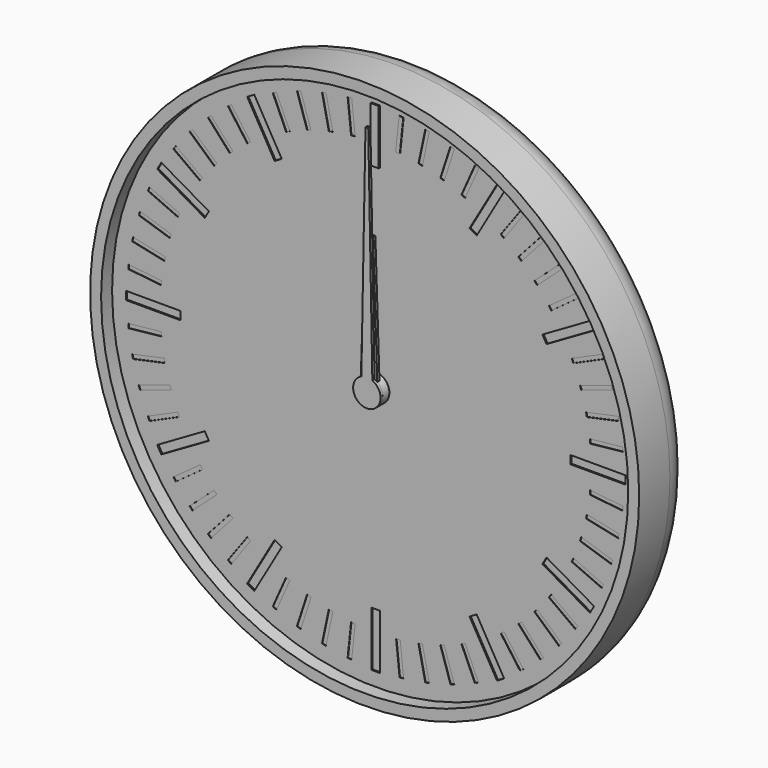
from build123d import *

# Parameters (mm, degrees)
F0_R      = 100
F1_DEPTH  = 24
F2_R      = 10
F3_T      = -4
F4_R      = 5
F4_R_2    = 3
F5_DEPTH  = 2
F6_DEPTH  = 19
F7_DEPTH  = 8
F9_DEPTH  = 4
F11_DEPTH = 4
F12_R     = 5
F12_R_2   = 3
F13_DEPTH = 2
F14_R     = 3
F15_DEPTH = 4
F17_DEPTH = 4
F18_R     = 3
F19_DEPTH = 2
F20_R     = 98
F20_R_2   = 5
F21_DEPTH = 1
F23_R     = 5
F23_R_2   = 3
F24_DEPTH = 2
F25_W     = 3
F25_H     = 20
F25_W_2   = 20
F25_H_2   = 3
F26_DEPTH = 0.5
F27_W     = 1.5
F27_H     = 12
F27_W_2   = 12
F27_H_2   = 1.5
F28_DEPTH = 0.2
F29_DEPTH = 1
F30_DEPTH = 0.4
F31_R     = 5
F31_R_2   = 3
F32_DEPTH = 5
F33_R     = 3
F34_DEPTH = 1
F36_DEPTH = 1


with BuildPart() as f1:
    # F0 (on Front) → F1 (new body)
    with BuildSketch(Plane.XZ):
        Circle(F0_R)
    extrude(amount=F1_DEPTH)

    # F2
    f2_edges = [f1.edges().sort_by_distance(p)[0] for p in [
        (-100, 0, 0),
    ]]
    fillet(f2_edges, radius=F2_R)

    # F3
    f3_openings = [f1.faces().sort_by_distance(p)[0] for p in [
        (0, -24, 0),
    ]]
    offset(amount=F3_T, openings=f3_openings)

    # F4 (on face) → F5 (join)
    with BuildSketch(Plane.XZ.offset(4)):
        Circle(F4_R)
        Circle(F4_R_2, mode=Mode.SUBTRACT)
        with Locations((40, 0)):
            Circle(F4_R)
        with Locations((40, 0)):
            Circle(F4_R_2, mode=Mode.SUBTRACT)
    extrude(amount=F5_DEPTH)


with BuildPart() as f6:
    # F6 (new): a face of the model
    f6_faces = [f1.part.faces().sort_by_distance(p)[0] for p in [
        (0, -4, 0),
    ]]
    extrude(f6_faces, amount=F6_DEPTH)

    # F8 (on face) → F9 (join)
    with BuildSketch(Plane.XZ.offset(6)):
        with BuildLine():
            ThreePointArc((9.2729637667, -1.3794085621), (9.3494561423, -0.6915886375), (9.375, 0))
            ThreePointArc((9.375, 0), (9.3494561423, 0.6915886375), (9.2729637667, 1.3794085621))
            ThreePointArc((9.2729637667, 1.3794085621), (8.9161548403, 2.8970343223), (8.3127812852, 4.3345463782))
            ThreePointArc((8.3127812852, 4.3345463782), (7.5845343223, 5.5104867402), (6.6911892658, 6.566476316))
            ThreePointArc((6.6911892658, 6.566476316), (5.5104867402, 7.5845343223), (4.1773988938, 8.3928519278))
            ThreePointArc((4.1773988938, 8.3928519278), (2.8970343223, 8.9161548403), (1.5536078905, 9.2453733036))
            ThreePointArc((1.5536078905, 9.2453733036), (0, 9.375), (-1.5536078905, 9.2453733036))
            ThreePointArc((-1.5536078905, 9.2453733036), (-2.8970343223, 8.9161548403), (-4.1773988938, 8.3928519278))
            ThreePointArc((-4.1773988938, 8.3928519278), (-5.5104867402, 7.5845343223), (-6.6911892658, 6.566476316))
            ThreePointArc((-6.6911892658, 6.566476316), (-7.5845343223, 5.5104867402), (-8.3127812852, 4.3345463782))
            ThreePointArc((-8.3127812852, 4.3345463782), (-8.9161548403, 2.8970343223), (-9.2729637667, 1.3794085621))
            ThreePointArc((-9.2729637667, 1.3794085621), (-9.375, 0), (-9.2729637667, -1.3794085621))
            ThreePointArc((-9.2729637667, -1.3794085621), (-8.9161548403, -2.8970343223), (-8.3127812852, -4.3345463782))
            ThreePointArc((-8.3127812852, -4.3345463782), (-7.5845343223, -5.5104867402), (-6.6911892658, -6.566476316))
            ThreePointArc((-6.6911892658, -6.566476316), (-5.5104867402, -7.5845343223), (-4.1773988938, -8.3928519278))
            ThreePointArc((-4.1773988938, -8.3928519278), (-2.8970343223, -8.9161548403), (-1.5536078905, -9.2453733036))
            ThreePointArc((-1.5536078905, -9.2453733036), (0, -9.375), (1.5536078905, -9.2453733036))
            ThreePointArc((1.5536078905, -9.2453733036), (2.8970343223, -8.9161548403), (4.1773988938, -8.3928519278))
            ThreePointArc((4.1773988938, -8.3928519278), (5.5104867402, -7.5845343223), (6.6911892658, -6.566476316))
            ThreePointArc((6.6911892658, -6.566476316), (7.5845343223, -5.5104867402), (8.3127812852, -4.3345463782))
            ThreePointArc((8.3127812852, -4.3345463782), (8.9161548403, -2.8970343223), (9.2729637667, -1.3794085621))
        make_face()
        with BuildLine():
            ThreePointArc((8.3127812852, 4.3345463782), (8.9161548403, 2.8970343223), (9.2729637667, 1.3794085621))
            Line((9.2729637667, 1.3794085621), (11.1823199426, 2.3946312492))
            Line((11.1823199426, 2.3946312492), (10.8182678729, 3.515068311))
            Line((10.8182678729, 3.515068311), (10.4542158031, 4.6355053728))
            Line((10.4542158031, 4.6355053728), (8.3127812852, 4.3345463782))
        make_face()
        with BuildLine():
            Line((11.1823199426, -2.3946312492), (9.2729637667, -1.3794085621))
            ThreePointArc((9.2729637667, -1.3794085621), (8.9161548403, -2.8970343223), (8.3127812852, -4.3345463782))
            Line((8.3127812852, -4.3345463782), (10.4542158031, -4.6355053728))
            Line((10.4542158031, -4.6355053728), (10.8182678729, -3.515068311))
            Line((10.8182678729, -3.515068311), (11.1823199426, -2.3946312492))
        make_face()
        with BuildLine():
            ThreePointArc((4.1773988938, 8.3928519278), (5.5104867402, 7.5845343223), (6.6911892658, 6.566476316))
            Line((6.6911892658, 6.566476316), (7.6391579371, 8.5101001246))
            Line((7.6391579371, 8.5101001246), (6.6860572448, 9.202568311))
            Line((6.6860572448, 9.202568311), (5.7329565525, 9.8950364974))
            Line((5.7329565525, 9.8950364974), (4.1773988938, 8.3928519278))
        make_face()
        with BuildLine():
            Line((7.6391579371, -8.5101001246), (6.6911892658, -6.566476316))
            ThreePointArc((6.6911892658, -6.566476316), (5.5104867402, -7.5845343223), (4.1773988938, -8.3928519278))
            Line((4.1773988938, -8.3928519278), (5.7329565525, -9.8950364974))
            Line((5.7329565525, -9.8950364974), (6.6860572448, -9.202568311))
            Line((6.6860572448, -9.202568311), (7.6391579371, -8.5101001246))
        make_face()
        with BuildLine():
            ThreePointArc((-1.5536078905, 9.2453733036), (0, 9.375), (1.5536078905, 9.2453733036))
            Line((1.5536078905, 9.2453733036), (1.1780972451, 11.375))
            Line((1.1780972451, 11.375), (0, 11.375))
            Line((0, 11.375), (-1.1780972451, 11.375))
            Line((-1.1780972451, 11.375), (-1.5536078905, 9.2453733036))
        make_face()
        with BuildLine():
            Line((1.1780972451, -11.375), (1.5536078905, -9.2453733036))
            ThreePointArc((1.5536078905, -9.2453733036), (0, -9.375), (-1.5536078905, -9.2453733036))
            Line((-1.5536078905, -9.2453733036), (-1.1780972451, -11.375))
            Line((-1.1780972451, -11.375), (0, -11.375))
            Line((0, -11.375), (1.1780972451, -11.375))
        make_face()
        with BuildLine():
            ThreePointArc((-6.6911892658, 6.566476316), (-5.5104867402, 7.5845343223), (-4.1773988938, 8.3928519278))
            Line((-4.1773988938, 8.3928519278), (-5.7329565525, 9.8950364974))
            Line((-5.7329565525, 9.8950364974), (-6.6860572448, 9.202568311))
            Line((-6.6860572448, 9.202568311), (-7.6391579371, 8.5101001246))
            Line((-7.6391579371, 8.5101001246), (-6.6911892658, 6.566476316))
        make_face()
        with BuildLine():
            Line((-5.7329565525, -9.8950364974), (-4.1773988938, -8.3928519278))
            ThreePointArc((-4.1773988938, -8.3928519278), (-5.5104867402, -7.5845343223), (-6.6911892658, -6.566476316))
            Line((-6.6911892658, -6.566476316), (-7.6391579371, -8.5101001246))
            Line((-7.6391579371, -8.5101001246), (-6.6860572448, -9.202568311))
            Line((-6.6860572448, -9.202568311), (-5.7329565525, -9.8950364974))
        make_face()
        with BuildLine():
            ThreePointArc((-9.2729637667, 1.3794085621), (-8.9161548403, 2.8970343223), (-8.3127812852, 4.3345463782))
            Line((-8.3127812852, 4.3345463782), (-10.4542158031, 4.6355053728))
            Line((-10.4542158031, 4.6355053728), (-10.8182678729, 3.515068311))
            Line((-10.8182678729, 3.515068311), (-11.1823199426, 2.3946312492))
            Line((-11.1823199426, 2.3946312492), (-9.2729637667, 1.3794085621))
        make_face()
        with BuildLine():
            Line((-10.4542158031, -4.6355053728), (-8.3127812852, -4.3345463782))
            ThreePointArc((-8.3127812852, -4.3345463782), (-8.9161548403, -2.8970343223), (-9.2729637667, -1.3794085621))
            Line((-9.2729637667, -1.3794085621), (-11.1823199426, -2.3946312492))
            Line((-11.1823199426, -2.3946312492), (-10.8182678729, -3.515068311))
            Line((-10.8182678729, -3.515068311), (-10.4542158031, -4.6355053728))
        make_face()
    extrude(amount=F9_DEPTH)

    # F35 (on face) → F36 (join)
    with BuildSketch(Plane.XZ.offset(23)):
        with BuildLine():
            ThreePointArc((-2, 4.582575695), (-2.7386127875, -4.1833001327), (5, 0))
            ThreePointArc((5, 0), (4.1833001327, 2.7386127875), (2, 4.582575695))
            ThreePointArc((2, 4.582575695), (0, 5), (-2, 4.582575695))
        make_face()
        with BuildLine():
            ThreePointArc((-2, 4.582575695), (0, 5), (2, 4.582575695))
            Line((2, 4.582575695), (0.5, 85))
            Line((0.5, 85), (0, 85))
            Line((0, 85), (-0.5, 85))
            Line((-0.5, 85), (-2, 4.582575695))
        make_face()
    extrude(amount=-F36_DEPTH)


with BuildPart() as f7:
    # F7 (new): a face of the model
    f7_faces = [f1.part.faces().sort_by_distance(p)[0] for p in [
        (40, -4, 0),
    ]]
    extrude(f7_faces, amount=F7_DEPTH)

    # F10 (on face) → F11 (join)
    with BuildSketch(Plane.XZ.offset(6)):
        with BuildLine():
            ThreePointArc((68.0829066802, -1.5381733945), (68.1144747006, -0.7693746225), (68.125, 0))
            ThreePointArc((68.125, 0), (68.1144747006, 0.7693746225), (68.0829066802, 1.5381733945))
            ThreePointArc((68.0829066802, 1.5381733945), (67.9709283072, 2.9398630294), (67.7890320221, 4.3342039956))
            ThreePointArc((67.7890320221, 4.3342039956), (67.5104012706, 5.8475163042), (67.1494235596, 7.3433252263))
            ThreePointArc((67.1494235596, 7.3433252263), (66.7484645208, 8.6911029668), (66.280643318, 10.0171558733))
            ThreePointArc((66.280643318, 10.0171558733), (65.6934659962, 11.4394680865), (65.0293803521, 12.8275385085))
            ThreePointArc((65.0293803521, 12.8275385085), (64.3569644814, 14.0625), (63.6236643925, 15.2623099717))
            ThreePointArc((63.6236643925, 15.2623099717), (62.7536029668, 16.5314602207), (61.815433119, 17.7511268046))
            ThreePointArc((61.815433119, 17.7511268046), (60.9009482166, 18.8192983038), (59.934217974, 19.8404278876))
            ThreePointArc((59.934217974, 19.8404278876), (58.8192983038, 20.9009482166), (57.6480467764, 21.8989056799))
            ThreePointArc((57.6480467764, 21.8989056799), (56.5314602207, 22.7536029668), (55.3735505752, 23.5514238999))
            ThreePointArc((55.3735505752, 23.5514238999), (54.0625, 24.3569644814), (52.709356105, 25.0895972944))
            ThreePointArc((52.709356105, 25.0895972944), (51.4394680865, 25.6934659962), (50.1409852457, 26.2331096755))
            ThreePointArc((50.1409852457, 26.2331096755), (48.6911029668, 26.7484645208), (47.2152055856, 27.1837531139))
            ThreePointArc((47.2152055856, 27.1837531139), (45.8475163042, 27.5104012706), (44.4652101991, 27.7682826779))
            ThreePointArc((44.4652101991, 27.7682826779), (42.9398630294, 27.9709283072), (41.4057159597, 28.0898484802))
            ThreePointArc((41.4057159597, 28.0898484802), (40, 28.125), (38.5942840403, 28.0898484802))
            ThreePointArc((38.5942840403, 28.0898484802), (37.0601369706, 27.9709283072), (35.5347898009, 27.7682826779))
            ThreePointArc((35.5347898009, 27.7682826779), (34.1524836958, 27.5104012706), (32.7847944144, 27.1837531139))
            ThreePointArc((32.7847944144, 27.1837531139), (31.3088970332, 26.7484645208), (29.8590147543, 26.2331096755))
            ThreePointArc((29.8590147543, 26.2331096755), (28.5605319135, 25.6934659962), (27.290643895, 25.0895972944))
            ThreePointArc((27.290643895, 25.0895972944), (25.9375, 24.3569644814), (24.6264494248, 23.5514238999))
            ThreePointArc((24.6264494248, 23.5514238999), (23.4685397793, 22.7536029668), (22.3519532236, 21.8989056799))
            ThreePointArc((22.3519532236, 21.8989056799), (21.1807016962, 20.9009482166), (20.065782026, 19.8404278876))
            ThreePointArc((20.065782026, 19.8404278876), (19.0990517834, 18.8192983038), (18.184566881, 17.7511268046))
            ThreePointArc((18.184566881, 17.7511268046), (17.2463970332, 16.5314602207), (16.3763356075, 15.2623099717))
            ThreePointArc((16.3763356075, 15.2623099717), (15.6430355186, 14.0625), (14.9706196479, 12.8275385085))
            ThreePointArc((14.9706196479, 12.8275385085), (14.3065340038, 11.4394680865), (13.719356682, 10.0171558733))
            ThreePointArc((13.719356682, 10.0171558733), (13.2515354792, 8.6911029668), (12.8505764404, 7.3433252263))
            ThreePointArc((12.8505764404, 7.3433252263), (12.4895987294, 5.8475163042), (12.2109679779, 4.3342039956))
            ThreePointArc((12.2109679779, 4.3342039956), (12.0290716928, 2.9398630294), (11.9170933198, 1.5381733945))
            ThreePointArc((11.9170933198, 1.5381733945), (11.875, 0), (11.9170933198, -1.5381733945))
            ThreePointArc((11.9170933198, -1.5381733945), (12.0290716928, -2.9398630294), (12.2109679779, -4.3342039956))
            ThreePointArc((12.2109679779, -4.3342039956), (12.4895987294, -5.8475163042), (12.8505764404, -7.3433252263))
            ThreePointArc((12.8505764404, -7.3433252263), (13.2515354792, -8.6911029668), (13.719356682, -10.0171558733))
            ThreePointArc((13.719356682, -10.0171558733), (14.3065340038, -11.4394680865), (14.9706196479, -12.8275385085))
            ThreePointArc((14.9706196479, -12.8275385085), (15.6430355186, -14.0625), (16.3763356075, -15.2623099717))
            ThreePointArc((16.3763356075, -15.2623099717), (17.2463970332, -16.5314602207), (18.184566881, -17.7511268046))
            ThreePointArc((18.184566881, -17.7511268046), (19.0990517834, -18.8192983038), (20.065782026, -19.8404278876))
            ThreePointArc((20.065782026, -19.8404278876), (21.1807016962, -20.9009482166), (22.3519532236, -21.8989056799))
            ThreePointArc((22.3519532236, -21.8989056799), (23.4685397793, -22.7536029668), (24.6264494248, -23.5514238999))
            ThreePointArc((24.6264494248, -23.5514238999), (25.9375, -24.3569644814), (27.290643895, -25.0895972944))
            ThreePointArc((27.290643895, -25.0895972944), (28.5605319135, -25.6934659962), (29.8590147543, -26.2331096755))
            ThreePointArc((29.8590147543, -26.2331096755), (31.3088970332, -26.7484645208), (32.7847944144, -27.1837531139))
            ThreePointArc((32.7847944144, -27.1837531139), (34.1524836958, -27.5104012706), (35.5347898009, -27.7682826779))
            ThreePointArc((35.5347898009, -27.7682826779), (37.0601369706, -27.9709283072), (38.5942840403, -28.0898484802))
            ThreePointArc((38.5942840403, -28.0898484802), (40, -28.125), (41.4057159597, -28.0898484802))
            ThreePointArc((41.4057159597, -28.0898484802), (42.9398630294, -27.9709283072), (44.4652101991, -27.7682826779))
            ThreePointArc((44.4652101991, -27.7682826779), (45.8475163042, -27.5104012706), (47.2152055856, -27.1837531139))
            ThreePointArc((47.2152055856, -27.1837531139), (48.6911029668, -26.7484645208), (50.1409852457, -26.2331096755))
            ThreePointArc((50.1409852457, -26.2331096755), (51.4394680865, -25.6934659962), (52.709356105, -25.0895972944))
            ThreePointArc((52.709356105, -25.0895972944), (54.0625, -24.3569644814), (55.3735505752, -23.5514238999))
            ThreePointArc((55.3735505752, -23.5514238999), (56.5314602207, -22.7536029668), (57.6480467764, -21.8989056799))
            ThreePointArc((57.6480467764, -21.8989056799), (58.8192983038, -20.9009482166), (59.934217974, -19.8404278876))
            ThreePointArc((59.934217974, -19.8404278876), (60.9009482166, -18.8192983038), (61.815433119, -17.7511268046))
            ThreePointArc((61.815433119, -17.7511268046), (62.7536029668, -16.5314602207), (63.6236643925, -15.2623099717))
            ThreePointArc((63.6236643925, -15.2623099717), (64.3569644814, -14.0625), (65.0293803521, -12.8275385085))
            ThreePointArc((65.0293803521, -12.8275385085), (65.6934659962, -11.4394680865), (66.280643318, -10.0171558733))
            ThreePointArc((66.280643318, -10.0171558733), (66.7484645208, -8.6911029668), (67.1494235596, -7.3433252263))
            ThreePointArc((67.1494235596, -7.3433252263), (67.5104012706, -5.8475163042), (67.7890320221, -4.3342039956))
            ThreePointArc((67.7890320221, -4.3342039956), (67.9709283072, -2.9398630294), (68.0829066802, -1.5381733945))
        make_face()
        with BuildLine():
            ThreePointArc((68.0829066802, 1.5381733945), (68.1144747006, 0.7693746225), (68.125, 0))
            ThreePointArc((68.125, 0), (68.1144747006, -0.7693746225), (68.0829066802, -1.5381733945))
            Line((68.0829066802, -1.5381733945), (70.125, -1.1780972451))
            Line((70.125, -1.1780972451), (70.125, 0))
            Line((70.125, 0), (70.125, 1.1780972451))
            Line((70.125, 1.1780972451), (68.0829066802, 1.5381733945))
        make_face()
        with BuildLine():
            ThreePointArc((67.1494235596, 7.3433252263), (67.5104012706, 5.8475163042), (67.7890320221, 4.3342039956))
            Line((67.7890320221, 4.3342039956), (69.7116366623, 5.1109866922))
            Line((69.7116366623, 5.1109866922), (69.4666964721, 6.2633396859))
            Line((69.4666964721, 6.2633396859), (69.2217562819, 7.4156926796))
            Line((69.2217562819, 7.4156926796), (67.1494235596, 7.3433252263))
        make_face()
        with BuildLine():
            Line((69.7116366623, -5.1109866922), (67.7890320221, -4.3342039956))
            ThreePointArc((67.7890320221, -4.3342039956), (67.5104012706, -5.8475163042), (67.1494235596, -7.3433252263))
            Line((67.1494235596, -7.3433252263), (69.2217562819, -7.4156926796))
            Line((69.2217562819, -7.4156926796), (69.4666964721, -6.2633396859))
            Line((69.4666964721, -6.2633396859), (69.7116366623, -5.1109866922))
        make_face()
        with BuildLine():
            ThreePointArc((65.0293803521, 12.8275385085), (65.6934659962, 11.4394680865), (66.280643318, 10.0171558733))
            Line((66.280643318, 10.0171558733), (67.9997322302, 11.1766959857))
            Line((67.9997322302, 11.1766959857), (67.5205569115, 12.2529413727))
            Line((67.5205569115, 12.2529413727), (67.0413815928, 13.3291867596))
            Line((67.0413815928, 13.3291867596), (65.0293803521, 12.8275385085))
        make_face()
        with BuildLine():
            Line((67.9997322302, -11.1766959857), (66.280643318, -10.0171558733))
            ThreePointArc((66.280643318, -10.0171558733), (65.6934659962, -11.4394680865), (65.0293803521, -12.8275385085))
            Line((65.0293803521, -12.8275385085), (67.0413815928, -13.3291867596))
            Line((67.0413815928, -13.3291867596), (67.5205569115, -12.2529413727))
            Line((67.5205569115, -12.2529413727), (67.9997322302, -11.1766959857))
        make_face()
        with BuildLine():
            ThreePointArc((61.815433119, 17.7511268046), (62.7536029668, 16.5314602207), (63.6236643925, 15.2623099717))
            Line((63.6236643925, 15.2623099717), (65.064105142, 16.753930033))
            Line((65.064105142, 16.753930033), (64.3716369555, 17.7070307253))
            Line((64.3716369555, 17.7070307253), (63.6791687691, 18.6601314176))
            Line((63.6791687691, 18.6601314176), (61.815433119, 17.7511268046))
        make_face()
        with BuildLine():
            Line((65.064105142, -16.753930033), (63.6236643925, -15.2623099717))
            ThreePointArc((63.6236643925, -15.2623099717), (62.7536029668, -16.5314602207), (61.815433119, -17.7511268046))
            Line((61.815433119, -17.7511268046), (63.6791687691, -18.6601314176))
            Line((63.6791687691, -18.6601314176), (64.3716369555, -17.7070307253))
            Line((64.3716369555, -17.7070307253), (65.064105142, -16.753930033))
        make_face()
        with BuildLine():
            ThreePointArc((57.6480467764, 21.8989056799), (58.8192983038, 20.9009482166), (59.934217974, 19.8404278876))
            Line((59.934217974, 19.8404278876), (61.0330563882, 21.5989369435))
            Line((61.0330563882, 21.5989369435), (60.1575595166, 22.3872378675))
            Line((60.1575595166, 22.3872378675), (59.282062645, 23.1755387915))
            Line((59.282062645, 23.1755387915), (57.6480467764, 21.8989056799))
        make_face()
        with BuildLine():
            Line((61.0330563882, -21.5989369435), (59.934217974, -19.8404278876))
            ThreePointArc((59.934217974, -19.8404278876), (58.8192983038, -20.9009482166), (57.6480467764, -21.8989056799))
            Line((57.6480467764, -21.8989056799), (59.282062645, -23.1755387915))
            Line((59.282062645, -23.1755387915), (60.1575595166, -22.3872378675))
            Line((60.1575595166, -22.3872378675), (61.0330563882, -21.5989369435))
        make_face()
        with BuildLine():
            ThreePointArc((52.709356105, 25.0895972944), (54.0625, 24.3569644814), (55.3735505752, 23.5514238999))
            Line((55.3735505752, 23.5514238999), (56.0827621424, 25.4999666665))
            Line((56.0827621424, 25.4999666665), (55.0625, 26.089015289))
            Line((55.0625, 26.089015289), (54.0422378576, 26.6780639116))
            Line((54.0422378576, 26.6780639116), (52.709356105, 25.0895972944))
        make_face()
        with BuildLine():
            Line((56.0827621424, -25.4999666665), (55.3735505752, -23.5514238999))
            ThreePointArc((55.3735505752, -23.5514238999), (54.0625, -24.3569644814), (52.709356105, -25.0895972944))
            Line((52.709356105, -25.0895972944), (54.0422378576, -26.6780639116))
            Line((54.0422378576, -26.6780639116), (55.0625, -26.089015289))
            Line((55.0625, -26.089015289), (56.0827621424, -25.4999666665))
        make_face()
        with BuildLine():
            ThreePointArc((47.2152055856, 27.1837531139), (48.6911029668, 26.7484645208), (50.1409852457, 26.2331096755))
            Line((50.1409852457, 26.2331096755), (50.4295740173, 28.2865254836))
            Line((50.4295740173, 28.2865254836), (49.3091369555, 28.6505775534))
            Line((49.3091369555, 28.6505775534), (48.1886998938, 29.0146296232))
            Line((48.1886998938, 29.0146296232), (47.2152055856, 27.1837531139))
        make_face()
        with BuildLine():
            Line((50.4295740173, -28.2865254836), (50.1409852457, -26.2331096755))
            ThreePointArc((50.1409852457, -26.2331096755), (48.6911029668, -26.7484645208), (47.2152055856, -27.1837531139))
            Line((47.2152055856, -27.1837531139), (48.1886998938, -29.0146296232))
            Line((48.1886998938, -29.0146296232), (49.3091369555, -28.6505775534))
            Line((49.3091369555, -28.6505775534), (50.4295740173, -28.2865254836))
        make_face()
        with BuildLine():
            ThreePointArc((41.4057159597, 28.0898484802), (42.9398630294, 27.9709283072), (44.4652101991, 27.7682826779))
            Line((44.4652101991, 27.7682826779), (44.3205634611, 29.8368274034))
            Line((44.3205634611, 29.8368274034), (43.1489199559, 29.959972098))
            Line((43.1489199559, 29.959972098), (41.9772764508, 30.0831167926))
            Line((41.9772764508, 30.0831167926), (41.4057159597, 28.0898484802))
        make_face()
        with BuildLine():
            Line((44.3205634611, -29.8368274034), (44.4652101991, -27.7682826779))
            ThreePointArc((44.4652101991, -27.7682826779), (42.9398630294, -27.9709283072), (41.4057159597, -28.0898484802))
            Line((41.4057159597, -28.0898484802), (41.9772764508, -30.0831167926))
            Line((41.9772764508, -30.0831167926), (43.1489199559, -29.959972098))
            Line((43.1489199559, -29.959972098), (44.3205634611, -29.8368274034))
        make_face()
        with BuildLine():
            ThreePointArc((35.5347898009, 27.7682826779), (37.0601369706, 27.9709283072), (38.5942840403, 28.0898484802))
            Line((38.5942840403, 28.0898484802), (38.0227235492, 30.0831167926))
            Line((38.0227235492, 30.0831167926), (36.8510800441, 29.959972098))
            Line((36.8510800441, 29.959972098), (35.6794365389, 29.8368274034))
            Line((35.6794365389, 29.8368274034), (35.5347898009, 27.7682826779))
        make_face()
        with BuildLine():
            Line((38.0227235492, -30.0831167926), (38.5942840403, -28.0898484802))
            ThreePointArc((38.5942840403, -28.0898484802), (37.0601369706, -27.9709283072), (35.5347898009, -27.7682826779))
            Line((35.5347898009, -27.7682826779), (35.6794365389, -29.8368274034))
            Line((35.6794365389, -29.8368274034), (36.8510800441, -29.959972098))
            Line((36.8510800441, -29.959972098), (38.0227235492, -30.0831167926))
        make_face()
        with BuildLine():
            ThreePointArc((29.8590147543, 26.2331096755), (31.3088970332, 26.7484645208), (32.7847944144, 27.1837531139))
            Line((32.7847944144, 27.1837531139), (31.8113001062, 29.0146296232))
            Line((31.8113001062, 29.0146296232), (30.6908630445, 28.6505775534))
            Line((30.6908630445, 28.6505775534), (29.5704259827, 28.2865254836))
            Line((29.5704259827, 28.2865254836), (29.8590147543, 26.2331096755))
        make_face()
        with BuildLine():
            Line((31.8113001062, -29.0146296232), (32.7847944144, -27.1837531139))
            ThreePointArc((32.7847944144, -27.1837531139), (31.3088970332, -26.7484645208), (29.8590147543, -26.2331096755))
            Line((29.8590147543, -26.2331096755), (29.5704259827, -28.2865254836))
            Line((29.5704259827, -28.2865254836), (30.6908630445, -28.6505775534))
            Line((30.6908630445, -28.6505775534), (31.8113001062, -29.0146296232))
        make_face()
        with BuildLine():
            ThreePointArc((24.6264494248, 23.5514238999), (25.9375, 24.3569644814), (27.290643895, 25.0895972944))
            Line((27.290643895, 25.0895972944), (25.9577621424, 26.6780639116))
            Line((25.9577621424, 26.6780639116), (24.9375, 26.089015289))
            Line((24.9375, 26.089015289), (23.9172378576, 25.4999666665))
            Line((23.9172378576, 25.4999666665), (24.6264494248, 23.5514238999))
        make_face()
        with BuildLine():
            Line((25.9577621424, -26.6780639116), (27.290643895, -25.0895972944))
            ThreePointArc((27.290643895, -25.0895972944), (25.9375, -24.3569644814), (24.6264494248, -23.5514238999))
            Line((24.6264494248, -23.5514238999), (23.9172378576, -25.4999666665))
            Line((23.9172378576, -25.4999666665), (24.9375, -26.089015289))
            Line((24.9375, -26.089015289), (25.9577621424, -26.6780639116))
        make_face()
        with BuildLine():
            ThreePointArc((20.065782026, 19.8404278876), (21.1807016962, 20.9009482166), (22.3519532236, 21.8989056799))
            Line((22.3519532236, 21.8989056799), (20.717937355, 23.1755387915))
            Line((20.717937355, 23.1755387915), (19.8424404834, 22.3872378675))
            Line((19.8424404834, 22.3872378675), (18.9669436118, 21.5989369435))
            Line((18.9669436118, 21.5989369435), (20.065782026, 19.8404278876))
        make_face()
        with BuildLine():
            Line((20.717937355, -23.1755387915), (22.3519532236, -21.8989056799))
            ThreePointArc((22.3519532236, -21.8989056799), (21.1807016962, -20.9009482166), (20.065782026, -19.8404278876))
            Line((20.065782026, -19.8404278876), (18.9669436118, -21.5989369435))
            Line((18.9669436118, -21.5989369435), (19.8424404834, -22.3872378675))
            Line((19.8424404834, -22.3872378675), (20.717937355, -23.1755387915))
        make_face()
        with BuildLine():
            ThreePointArc((16.3763356075, 15.2623099717), (17.2463970332, 16.5314602207), (18.184566881, 17.7511268046))
            Line((18.184566881, 17.7511268046), (16.3208312309, 18.6601314176))
            Line((16.3208312309, 18.6601314176), (15.6283630445, 17.7070307253))
            Line((15.6283630445, 17.7070307253), (14.935894858, 16.753930033))
            Line((14.935894858, 16.753930033), (16.3763356075, 15.2623099717))
        make_face()
        with BuildLine():
            Line((16.3208312309, -18.6601314176), (18.184566881, -17.7511268046))
            ThreePointArc((18.184566881, -17.7511268046), (17.2463970332, -16.5314602207), (16.3763356075, -15.2623099717))
            Line((16.3763356075, -15.2623099717), (14.935894858, -16.753930033))
            Line((14.935894858, -16.753930033), (15.6283630445, -17.7070307253))
            Line((15.6283630445, -17.7070307253), (16.3208312309, -18.6601314176))
        make_face()
        with BuildLine():
            ThreePointArc((13.719356682, 10.0171558733), (14.3065340038, 11.4394680865), (14.9706196479, 12.8275385085))
            Line((14.9706196479, 12.8275385085), (12.9586184072, 13.3291867596))
            Line((12.9586184072, 13.3291867596), (12.4794430885, 12.2529413727))
            Line((12.4794430885, 12.2529413727), (12.0002677698, 11.1766959857))
            Line((12.0002677698, 11.1766959857), (13.719356682, 10.0171558733))
        make_face()
        with BuildLine():
            Line((12.9586184072, -13.3291867596), (14.9706196479, -12.8275385085))
            ThreePointArc((14.9706196479, -12.8275385085), (14.3065340038, -11.4394680865), (13.719356682, -10.0171558733))
            Line((13.719356682, -10.0171558733), (12.0002677698, -11.1766959857))
            Line((12.0002677698, -11.1766959857), (12.4794430885, -12.2529413727))
            Line((12.4794430885, -12.2529413727), (12.9586184072, -13.3291867596))
        make_face()
        with BuildLine():
            ThreePointArc((12.2109679779, 4.3342039956), (12.4895987294, 5.8475163042), (12.8505764404, 7.3433252263))
            Line((12.8505764404, 7.3433252263), (10.7782437181, 7.4156926796))
            Line((10.7782437181, 7.4156926796), (10.5333035279, 6.2633396859))
            Line((10.5333035279, 6.2633396859), (10.2883633377, 5.1109866922))
            Line((10.2883633377, 5.1109866922), (12.2109679779, 4.3342039956))
        make_face()
        with BuildLine():
            Line((10.7782437181, -7.4156926796), (12.8505764404, -7.3433252263))
            ThreePointArc((12.8505764404, -7.3433252263), (12.4895987294, -5.8475163042), (12.2109679779, -4.3342039956))
            Line((12.2109679779, -4.3342039956), (10.2883633377, -5.1109866922))
            Line((10.2883633377, -5.1109866922), (10.5333035279, -6.2633396859))
            Line((10.5333035279, -6.2633396859), (10.7782437181, -7.4156926796))
        make_face()
        with BuildLine():
            ThreePointArc((11.9170933198, -1.5381733945), (11.875, 0), (11.9170933198, 1.5381733945))
            Line((11.9170933198, 1.5381733945), (9.875, 1.1780972451))
            Line((9.875, 1.1780972451), (9.875, 0))
            Line((9.875, 0), (9.875, -1.1780972451))
            Line((9.875, -1.1780972451), (11.9170933198, -1.5381733945))
        make_face()
    extrude(amount=F11_DEPTH)

    # F16 (on face) → F17 (join)
    with BuildSketch(Plane.XZ.offset(12)):
        with BuildLine():
            ThreePointArc((47.4288750323, -1.0304444454), (47.4821976298, -0.5164480894), (47.5, 0))
            ThreePointArc((47.5, 0), (47.4821976298, 0.5164480894), (47.4288750323, 1.0304444454))
            ThreePointArc((47.4288750323, 1.0304444454), (47.1329238722, 2.3176274578), (46.6157661985, 3.532936117))
            ThreePointArc((46.6157661985, 3.532936117), (46.0676274578, 4.4083893922), (45.4044061018, 5.2002302532))
            ThreePointArc((45.4044061018, 5.2002302532), (44.4083893922, 6.0676274578), (43.2756595386, 6.7468551628))
            ThreePointArc((43.2756595386, 6.7468551628), (42.3176274578, 7.1329238722), (41.3156377295, 7.3837048536))
            ThreePointArc((41.3156377295, 7.3837048536), (40, 7.5), (38.6843622705, 7.3837048536))
            ThreePointArc((38.6843622705, 7.3837048536), (37.6823725422, 7.1329238722), (36.7243404614, 6.7468551628))
            ThreePointArc((36.7243404614, 6.7468551628), (35.5916106078, 6.0676274578), (34.5955938982, 5.2002302532))
            ThreePointArc((34.5955938982, 5.2002302532), (33.9323725422, 4.4083893922), (33.3842338015, 3.532936117))
            ThreePointArc((33.3842338015, 3.532936117), (32.8670761278, 2.3176274578), (32.5711249677, 1.0304444454))
            ThreePointArc((32.5711249677, 1.0304444454), (32.5, 0), (32.5711249677, -1.0304444454))
            ThreePointArc((32.5711249677, -1.0304444454), (32.8670761278, -2.3176274578), (33.3842338015, -3.532936117))
            ThreePointArc((33.3842338015, -3.532936117), (33.9323725422, -4.4083893922), (34.5955938982, -5.2002302532))
            ThreePointArc((34.5955938982, -5.2002302532), (35.5916106078, -6.0676274578), (36.7243404614, -6.7468551628))
            ThreePointArc((36.7243404614, -6.7468551628), (37.6823725422, -7.1329238722), (38.6843622705, -7.3837048536))
            ThreePointArc((38.6843622705, -7.3837048536), (40, -7.5), (41.3156377295, -7.3837048536))
            ThreePointArc((41.3156377295, -7.3837048536), (42.3176274578, -7.1329238722), (43.2756595386, -6.7468551628))
            ThreePointArc((43.2756595386, -6.7468551628), (44.4083893922, -6.0676274578), (45.4044061018, -5.2002302532))
            ThreePointArc((45.4044061018, -5.2002302532), (46.0676274578, -4.4083893922), (46.6157661985, -3.532936117))
            ThreePointArc((46.6157661985, -3.532936117), (47.1329238722, -2.3176274578), (47.4288750323, -1.0304444454))
        make_face()
        with BuildLine():
            ThreePointArc((46.6157661985, 3.532936117), (47.1329238722, 2.3176274578), (47.4288750323, 1.0304444454))
            Line((47.4288750323, 1.0304444454), (49.3262785606, 2.0393117971))
            Line((49.3262785606, 2.0393117971), (48.743795249, 3.832011096))
            Line((48.743795249, 3.832011096), (46.6157661985, 3.532936117))
        make_face()
        with BuildLine():
            Line((49.3262785606, -2.0393117971), (47.4288750323, -1.0304444454))
            ThreePointArc((47.4288750323, -1.0304444454), (47.1329238722, -2.3176274578), (46.6157661985, -3.532936117))
            Line((46.6157661985, -3.532936117), (48.743795249, -3.832011096))
            Line((48.743795249, -3.832011096), (49.3262785606, -2.0393117971))
        make_face()
        with BuildLine():
            ThreePointArc((43.2756595386, 6.7468551628), (44.4083893922, 6.0676274578), (45.4044061018, 5.2002302532))
            Line((45.4044061018, 5.2002302532), (46.3464404506, 7.1316868974))
            Line((46.3464404506, 7.1316868974), (44.8214793429, 8.2396359957))
            Line((44.8214793429, 8.2396359957), (43.2756595386, 6.7468551628))
        make_face()
        with BuildLine():
            Line((46.3464404506, -7.1316868974), (45.4044061018, -5.2002302532))
            ThreePointArc((45.4044061018, -5.2002302532), (44.4083893922, -6.0676274578), (43.2756595386, -6.7468551628))
            Line((43.2756595386, -6.7468551628), (44.8214793429, -8.2396359957))
            Line((44.8214793429, -8.2396359957), (46.3464404506, -7.1316868974))
        make_face()
        with BuildLine():
            ThreePointArc((38.6843622705, 7.3837048536), (40, 7.5), (41.3156377295, 7.3837048536))
            Line((41.3156377295, 7.3837048536), (40.9424777961, 9.5))
            Line((40.9424777961, 9.5), (39.0575222039, 9.5))
            Line((39.0575222039, 9.5), (38.6843622705, 7.3837048536))
        make_face()
        with BuildLine():
            Line((40.9424777961, -9.5), (41.3156377295, -7.3837048536))
            ThreePointArc((41.3156377295, -7.3837048536), (40, -7.5), (38.6843622705, -7.3837048536))
            Line((38.6843622705, -7.3837048536), (39.0575222039, -9.5))
            Line((39.0575222039, -9.5), (40.9424777961, -9.5))
        make_face()
        with BuildLine():
            ThreePointArc((34.5955938982, 5.2002302532), (35.5916106078, 6.0676274578), (36.7243404614, 6.7468551628))
            Line((36.7243404614, 6.7468551628), (35.1785206571, 8.2396359957))
            Line((35.1785206571, 8.2396359957), (33.6535595494, 7.1316868974))
            Line((33.6535595494, 7.1316868974), (34.5955938982, 5.2002302532))
        make_face()
        with BuildLine():
            Line((35.1785206571, -8.2396359957), (36.7243404614, -6.7468551628))
            ThreePointArc((36.7243404614, -6.7468551628), (35.5916106078, -6.0676274578), (34.5955938982, -5.2002302532))
            Line((34.5955938982, -5.2002302532), (33.6535595494, -7.1316868974))
            Line((33.6535595494, -7.1316868974), (35.1785206571, -8.2396359957))
        make_face()
        with BuildLine():
            ThreePointArc((32.5711249677, 1.0304444454), (32.8670761278, 2.3176274578), (33.3842338015, 3.532936117))
            Line((33.3842338015, 3.532936117), (31.256204751, 3.832011096))
            Line((31.256204751, 3.832011096), (30.6737214394, 2.0393117971))
            Line((30.6737214394, 2.0393117971), (32.5711249677, 1.0304444454))
        make_face()
        with BuildLine():
            Line((31.256204751, -3.832011096), (33.3842338015, -3.532936117))
            ThreePointArc((33.3842338015, -3.532936117), (32.8670761278, -2.3176274578), (32.5711249677, -1.0304444454))
            Line((32.5711249677, -1.0304444454), (30.6737214394, -2.0393117971))
            Line((30.6737214394, -2.0393117971), (31.256204751, -3.832011096))
        make_face()
    extrude(amount=F17_DEPTH)

    # F18 (on face) → F19 (join)
    with BuildSketch(Plane.XZ.offset(16)):
        with Locations((40, 0)):
            Circle(F18_R)
    extrude(amount=F19_DEPTH)


with BuildPart() as f13:
    # F12 (on face) → F13 (new body)
    with BuildSketch(Plane.XZ.offset(10)):
        Circle(F12_R)
        Circle(F12_R_2, mode=Mode.SUBTRACT)
    extrude(amount=F13_DEPTH)

    # F14 (on face) → F15 (join)
    with BuildSketch(Plane.XZ.offset(12)):
        with BuildLine():
            ThreePointArc((29.9718156995, -1.3001014101), (29.9929530972, -0.6502034357), (30, 0))
            ThreePointArc((30, 0), (29.9929530972, 0.6502034357), (29.9718156995, 1.3001014101))
            ThreePointArc((29.9718156995, 1.3001014101), (29.907520012, 2.3537728718), (29.8061935814, 3.4045299509))
            ThreePointArc((29.8061935814, 3.4045299509), (29.6306502179, 4.6930339512), (29.3994322443, 5.9727199596))
            ThreePointArc((29.3994322443, 5.9727199596), (29.1710976119, 7.0033609157), (28.9066440563, 8.0253304855))
            ThreePointArc((28.9066440563, 8.0253304855), (28.5316954889, 9.2705098312), (28.1031371961, 10.4982703213))
            ThreePointArc((28.1031371961, 10.4982703213), (27.7163859753, 11.480502971), (27.2953170189, 12.448520749))
            ThreePointArc((27.2953170189, 12.448520749), (26.7301957257, 13.6197149922), (26.1148496411, 14.765318426))
            ThreePointArc((26.1148496411, 14.765318426), (25.5792049306, 15.6749569415), (25.0118886885, 16.5651871174))
            ThreePointArc((25.0118886885, 16.5651871174), (24.2705098312, 17.6335575688), (23.4835278178, 18.6687953878))
            ThreePointArc((23.4835278178, 18.6687953878), (22.812178968, 19.4834414499), (22.1125846489, 20.2739636023))
            ThreePointArc((22.1125846489, 20.2739636023), (21.2132034356, 21.2132034356), (20.2739636023, 22.1125846489))
            ThreePointArc((20.2739636023, 22.1125846489), (19.4834414499, 22.812178968), (18.6687953878, 23.4835278178))
            ThreePointArc((18.6687953878, 23.4835278178), (17.6335575688, 24.2705098312), (16.5651871174, 25.0118886885))
            ThreePointArc((16.5651871174, 25.0118886885), (15.6749569415, 25.5792049306), (14.765318426, 26.1148496411))
            ThreePointArc((14.765318426, 26.1148496411), (13.6197149922, 26.7301957257), (12.448520749, 27.2953170189))
            ThreePointArc((12.448520749, 27.2953170189), (11.480502971, 27.7163859753), (10.4982703213, 28.1031371961))
            ThreePointArc((10.4982703213, 28.1031371961), (9.2705098312, 28.5316954889), (8.0253304855, 28.9066440563))
            ThreePointArc((8.0253304855, 28.9066440563), (7.0033609157, 29.1710976119), (5.9727199596, 29.3994322443))
            ThreePointArc((5.9727199596, 29.3994322443), (4.6930339512, 29.6306502179), (3.4045299509, 29.8061935814))
            ThreePointArc((3.4045299509, 29.8061935814), (2.3537728718, 29.907520012), (1.3001014101, 29.9718156995))
            ThreePointArc((1.3001014101, 29.9718156995), (0, 30), (-1.3001014101, 29.9718156995))
            ThreePointArc((-1.3001014101, 29.9718156995), (-2.3537728718, 29.907520012), (-3.4045299509, 29.8061935814))
            ThreePointArc((-3.4045299509, 29.8061935814), (-4.6930339512, 29.6306502179), (-5.9727199596, 29.3994322443))
            ThreePointArc((-5.9727199596, 29.3994322443), (-7.0033609157, 29.1710976119), (-8.0253304855, 28.9066440563))
            ThreePointArc((-8.0253304855, 28.9066440563), (-9.2705098312, 28.5316954889), (-10.4982703213, 28.1031371961))
            ThreePointArc((-10.4982703213, 28.1031371961), (-11.480502971, 27.7163859753), (-12.448520749, 27.2953170189))
            ThreePointArc((-12.448520749, 27.2953170189), (-13.6197149922, 26.7301957257), (-14.765318426, 26.1148496411))
            ThreePointArc((-14.765318426, 26.1148496411), (-15.6749569415, 25.5792049306), (-16.5651871174, 25.0118886885))
            ThreePointArc((-16.5651871174, 25.0118886885), (-17.6335575688, 24.2705098312), (-18.6687953878, 23.4835278178))
            ThreePointArc((-18.6687953878, 23.4835278178), (-19.4834414499, 22.812178968), (-20.2739636023, 22.1125846489))
            ThreePointArc((-20.2739636023, 22.1125846489), (-21.2132034356, 21.2132034356), (-22.1125846489, 20.2739636023))
            ThreePointArc((-22.1125846489, 20.2739636023), (-22.812178968, 19.4834414499), (-23.4835278178, 18.6687953878))
            ThreePointArc((-23.4835278178, 18.6687953878), (-24.2705098312, 17.6335575688), (-25.0118886885, 16.5651871174))
            ThreePointArc((-25.0118886885, 16.5651871174), (-25.5792049306, 15.6749569415), (-26.1148496411, 14.765318426))
            ThreePointArc((-26.1148496411, 14.765318426), (-26.7301957257, 13.6197149922), (-27.2953170189, 12.448520749))
            ThreePointArc((-27.2953170189, 12.448520749), (-27.7163859753, 11.480502971), (-28.1031371961, 10.4982703213))
            ThreePointArc((-28.1031371961, 10.4982703213), (-28.5316954889, 9.2705098312), (-28.9066440563, 8.0253304855))
            ThreePointArc((-28.9066440563, 8.0253304855), (-29.1710976119, 7.0033609157), (-29.3994322443, 5.9727199596))
            ThreePointArc((-29.3994322443, 5.9727199596), (-29.6306502179, 4.6930339512), (-29.8061935814, 3.4045299509))
            ThreePointArc((-29.8061935814, 3.4045299509), (-29.907520012, 2.3537728718), (-29.9718156995, 1.3001014101))
            ThreePointArc((-29.9718156995, 1.3001014101), (-30, 0), (-29.9718156995, -1.3001014101))
            ThreePointArc((-29.9718156995, -1.3001014101), (-29.907520012, -2.3537728718), (-29.8061935814, -3.4045299509))
            ThreePointArc((-29.8061935814, -3.4045299509), (-29.6306502179, -4.6930339512), (-29.3994322443, -5.9727199596))
            ThreePointArc((-29.3994322443, -5.9727199596), (-29.1710976119, -7.0033609157), (-28.9066440563, -8.0253304855))
            ThreePointArc((-28.9066440563, -8.0253304855), (-28.5316954889, -9.2705098312), (-28.1031371961, -10.4982703213))
            ThreePointArc((-28.1031371961, -10.4982703213), (-27.7163859753, -11.480502971), (-27.2953170189, -12.448520749))
            ThreePointArc((-27.2953170189, -12.448520749), (-26.7301957257, -13.6197149922), (-26.1148496411, -14.765318426))
            ThreePointArc((-26.1148496411, -14.765318426), (-25.5792049306, -15.6749569415), (-25.0118886885, -16.5651871174))
            ThreePointArc((-25.0118886885, -16.5651871174), (-24.2705098312, -17.6335575688), (-23.4835278178, -18.6687953878))
            ThreePointArc((-23.4835278178, -18.6687953878), (-22.812178968, -19.4834414499), (-22.1125846489, -20.2739636023))
            ThreePointArc((-22.1125846489, -20.2739636023), (-21.2132034356, -21.2132034356), (-20.2739636023, -22.1125846489))
            ThreePointArc((-20.2739636023, -22.1125846489), (-19.4834414499, -22.812178968), (-18.6687953878, -23.4835278178))
            ThreePointArc((-18.6687953878, -23.4835278178), (-17.6335575688, -24.2705098312), (-16.5651871174, -25.0118886885))
            ThreePointArc((-16.5651871174, -25.0118886885), (-15.6749569415, -25.5792049306), (-14.765318426, -26.1148496411))
            ThreePointArc((-14.765318426, -26.1148496411), (-13.6197149922, -26.7301957257), (-12.448520749, -27.2953170189))
            ThreePointArc((-12.448520749, -27.2953170189), (-11.480502971, -27.7163859753), (-10.4982703213, -28.1031371961))
            ThreePointArc((-10.4982703213, -28.1031371961), (-9.2705098312, -28.5316954889), (-8.0253304855, -28.9066440563))
            ThreePointArc((-8.0253304855, -28.9066440563), (-7.0033609157, -29.1710976119), (-5.9727199596, -29.3994322443))
            ThreePointArc((-5.9727199596, -29.3994322443), (-4.6930339512, -29.6306502179), (-3.4045299509, -29.8061935814))
            ThreePointArc((-3.4045299509, -29.8061935814), (-2.3537728718, -29.907520012), (-1.3001014101, -29.9718156995))
            ThreePointArc((-1.3001014101, -29.9718156995), (0, -30), (1.3001014101, -29.9718156995))
            ThreePointArc((1.3001014101, -29.9718156995), (2.3537728718, -29.907520012), (3.4045299509, -29.8061935814))
            ThreePointArc((3.4045299509, -29.8061935814), (4.6930339512, -29.6306502179), (5.9727199596, -29.3994322443))
            ThreePointArc((5.9727199596, -29.3994322443), (7.0033609157, -29.1710976119), (8.0253304855, -28.9066440563))
            ThreePointArc((8.0253304855, -28.9066440563), (9.2705098312, -28.5316954889), (10.4982703213, -28.1031371961))
            ThreePointArc((10.4982703213, -28.1031371961), (11.480502971, -27.7163859753), (12.448520749, -27.2953170189))
            ThreePointArc((12.448520749, -27.2953170189), (13.6197149922, -26.7301957257), (14.765318426, -26.1148496411))
            ThreePointArc((14.765318426, -26.1148496411), (15.6749569415, -25.5792049306), (16.5651871174, -25.0118886885))
            ThreePointArc((16.5651871174, -25.0118886885), (17.6335575688, -24.2705098312), (18.6687953878, -23.4835278178))
            ThreePointArc((18.6687953878, -23.4835278178), (19.4834414499, -22.812178968), (20.2739636023, -22.1125846489))
            ThreePointArc((20.2739636023, -22.1125846489), (21.2132034356, -21.2132034356), (22.1125846489, -20.2739636023))
            ThreePointArc((22.1125846489, -20.2739636023), (22.812178968, -19.4834414499), (23.4835278178, -18.6687953878))
            ThreePointArc((23.4835278178, -18.6687953878), (24.2705098312, -17.6335575688), (25.0118886885, -16.5651871174))
            ThreePointArc((25.0118886885, -16.5651871174), (25.5792049306, -15.6749569415), (26.1148496411, -14.765318426))
            ThreePointArc((26.1148496411, -14.765318426), (26.7301957257, -13.6197149922), (27.2953170189, -12.448520749))
            ThreePointArc((27.2953170189, -12.448520749), (27.7163859753, -11.480502971), (28.1031371961, -10.4982703213))
            ThreePointArc((28.1031371961, -10.4982703213), (28.5316954889, -9.2705098312), (28.9066440563, -8.0253304855))
            ThreePointArc((28.9066440563, -8.0253304855), (29.1710976119, -7.0033609157), (29.3994322443, -5.9727199596))
            ThreePointArc((29.3994322443, -5.9727199596), (29.6306502179, -4.6930339512), (29.8061935814, -3.4045299509))
            ThreePointArc((29.8061935814, -3.4045299509), (29.907520012, -2.3537728718), (29.9718156995, -1.3001014101))
        make_face()
        Circle(F14_R, mode=Mode.SUBTRACT)
        with BuildLine():
            ThreePointArc((29.9718156995, 1.3001014101), (29.9929530972, 0.6502034357), (30, 0))
            ThreePointArc((30, 0), (29.9929530972, -0.6502034357), (29.9718156995, -1.3001014101))
            Line((29.9718156995, -1.3001014101), (32, -0.9424777961))
            Line((32, -0.9424777961), (32, 0))
            Line((32, 0), (32, 0.9424777961))
            Line((32, 0.9424777961), (29.9718156995, 1.3001014101))
        make_face()
        with BuildLine():
            ThreePointArc((29.3994322443, 5.9727199596), (29.6306502179, 4.6930339512), (29.8061935814, 3.4045299509))
            Line((29.8061935814, 3.4045299509), (31.7534629089, 4.0750285508))
            Line((31.7534629089, 4.0750285508), (31.606026899, 5.0059028813))
            Line((31.606026899, 5.0059028813), (31.4585908892, 5.9367772117))
            Line((31.4585908892, 5.9367772117), (29.3994322443, 5.9727199596))
        make_face()
        with BuildLine():
            Line((31.7534629089, -4.0750285508), (29.8061935814, -3.4045299509))
            ThreePointArc((29.8061935814, -3.4045299509), (29.6306502179, -4.6930339512), (29.3994322443, -5.9727199596))
            Line((29.3994322443, -5.9727199596), (31.4585908892, -5.9367772117))
            Line((31.4585908892, -5.9367772117), (31.606026899, -5.0059028813))
            Line((31.606026899, -5.0059028813), (31.7534629089, -4.0750285508))
        make_face()
        with BuildLine():
            ThreePointArc((28.1031371961, 10.4982703213), (28.5316954889, 9.2705098312), (28.9066440563, 8.0253304855))
            Line((28.9066440563, 8.0253304855), (30.7250501773, 8.9921941706))
            Line((30.7250501773, 8.9921941706), (30.4338085214, 9.88854382))
            Line((30.4338085214, 9.88854382), (30.1425668656, 10.7848934694))
            Line((30.1425668656, 10.7848934694), (28.1031371961, 10.4982703213))
        make_face()
        with BuildLine():
            Line((30.7250501773, -8.9921941706), (28.9066440563, -8.0253304855))
            ThreePointArc((28.9066440563, -8.0253304855), (28.5316954889, -9.2705098312), (28.1031371961, -10.4982703213))
            Line((28.1031371961, -10.4982703213), (30.1425668656, -10.7848934694))
            Line((30.1425668656, -10.7848934694), (30.4338085214, -9.88854382))
            Line((30.4338085214, -9.88854382), (30.7250501773, -8.9921941706))
        make_face()
        with BuildLine():
            ThreePointArc((26.1148496411, 14.765318426), (26.7301957257, 13.6197149922), (27.2953170189, 12.448520749))
            Line((27.2953170189, 12.448520749), (28.9400847397, 13.6879421265))
            Line((28.9400847397, 13.6879421265), (28.512208774, 14.5276959917))
            Line((28.512208774, 14.5276959917), (28.0843328084, 15.3674498569))
            Line((28.0843328084, 15.3674498569), (26.1148496411, 14.765318426))
        make_face()
        with BuildLine():
            Line((28.9400847397, -13.6879421265), (27.2953170189, -12.448520749))
            ThreePointArc((27.2953170189, -12.448520749), (26.7301957257, -13.6197149922), (26.1148496411, -14.765318426))
            Line((26.1148496411, -14.765318426), (28.0843328084, -15.3674498569))
            Line((28.0843328084, -15.3674498569), (28.512208774, -14.5276959917))
            Line((28.512208774, -14.5276959917), (28.9400847397, -13.6879421265))
        make_face()
        with BuildLine():
            ThreePointArc((23.4835278178, 18.6687953878), (24.2705098312, 17.6335575688), (25.0118886885, 16.5651871174))
            Line((25.0118886885, 16.5651871174), (26.4425183691, 18.0466475195))
            Line((26.4425183691, 18.0466475195), (25.88854382, 18.8091280734))
            Line((25.88854382, 18.8091280734), (25.3345692709, 19.5716086272))
            Line((25.3345692709, 19.5716086272), (23.4835278178, 18.6687953878))
        make_face()
        with BuildLine():
            Line((26.4425183691, -18.0466475195), (25.0118886885, -16.5651871174))
            ThreePointArc((25.0118886885, -16.5651871174), (24.2705098312, -17.6335575688), (23.4835278178, -18.6687953878))
            Line((23.4835278178, -18.6687953878), (25.3345692709, -19.5716086272))
            Line((25.3345692709, -19.5716086272), (25.88854382, -18.8091280734))
            Line((25.88854382, -18.8091280734), (26.4425183691, -18.0466475195))
        make_face()
        with BuildLine():
            ThreePointArc((20.2739636023, 22.1125846489), (21.2132034356, 21.2132034356), (22.1125846489, 20.2739636023))
            Line((22.1125846489, 20.2739636023), (23.2938494387, 21.9609845572))
            Line((23.2938494387, 21.9609845572), (22.627416998, 22.627416998))
            Line((22.627416998, 22.627416998), (21.9609845572, 23.2938494387))
            Line((21.9609845572, 23.2938494387), (20.2739636023, 22.1125846489))
        make_face()
        with BuildLine():
            Line((23.2938494387, -21.9609845572), (22.1125846489, -20.2739636023))
            ThreePointArc((22.1125846489, -20.2739636023), (21.2132034356, -21.2132034356), (20.2739636023, -22.1125846489))
            Line((20.2739636023, -22.1125846489), (21.9609845572, -23.2938494387))
            Line((21.9609845572, -23.2938494387), (22.627416998, -22.627416998))
            Line((22.627416998, -22.627416998), (23.2938494387, -21.9609845572))
        make_face()
        with BuildLine():
            ThreePointArc((16.5651871174, 25.0118886885), (17.6335575688, 24.2705098312), (18.6687953878, 23.4835278178))
            Line((18.6687953878, 23.4835278178), (19.5716086272, 25.3345692709))
            Line((19.5716086272, 25.3345692709), (18.8091280734, 25.88854382))
            Line((18.8091280734, 25.88854382), (18.0466475195, 26.4425183691))
            Line((18.0466475195, 26.4425183691), (16.5651871174, 25.0118886885))
        make_face()
        with BuildLine():
            Line((19.5716086272, -25.3345692709), (18.6687953878, -23.4835278178))
            ThreePointArc((18.6687953878, -23.4835278178), (17.6335575688, -24.2705098312), (16.5651871174, -25.0118886885))
            Line((16.5651871174, -25.0118886885), (18.0466475195, -26.4425183691))
            Line((18.0466475195, -26.4425183691), (18.8091280734, -25.88854382))
            Line((18.8091280734, -25.88854382), (19.5716086272, -25.3345692709))
        make_face()
        with BuildLine():
            ThreePointArc((12.448520749, 27.2953170189), (13.6197149922, 26.7301957257), (14.765318426, 26.1148496411))
            Line((14.765318426, 26.1148496411), (15.3674498569, 28.0843328084))
            Line((15.3674498569, 28.0843328084), (14.5276959917, 28.512208774))
            Line((14.5276959917, 28.512208774), (13.6879421265, 28.9400847397))
            Line((13.6879421265, 28.9400847397), (12.448520749, 27.2953170189))
        make_face()
        with BuildLine():
            Line((15.3674498569, -28.0843328084), (14.765318426, -26.1148496411))
            ThreePointArc((14.765318426, -26.1148496411), (13.6197149922, -26.7301957257), (12.448520749, -27.2953170189))
            Line((12.448520749, -27.2953170189), (13.6879421265, -28.9400847397))
            Line((13.6879421265, -28.9400847397), (14.5276959917, -28.512208774))
            Line((14.5276959917, -28.512208774), (15.3674498569, -28.0843328084))
        make_face()
        with BuildLine():
            ThreePointArc((8.0253304855, 28.9066440563), (9.2705098312, 28.5316954889), (10.4982703213, 28.1031371961))
            Line((10.4982703213, 28.1031371961), (10.7848934694, 30.1425668656))
            Line((10.7848934694, 30.1425668656), (9.88854382, 30.4338085214))
            Line((9.88854382, 30.4338085214), (8.9921941706, 30.7250501773))
            Line((8.9921941706, 30.7250501773), (8.0253304855, 28.9066440563))
        make_face()
        with BuildLine():
            Line((10.7848934694, -30.1425668656), (10.4982703213, -28.1031371961))
            ThreePointArc((10.4982703213, -28.1031371961), (9.2705098312, -28.5316954889), (8.0253304855, -28.9066440563))
            Line((8.0253304855, -28.9066440563), (8.9921941706, -30.7250501773))
            Line((8.9921941706, -30.7250501773), (9.88854382, -30.4338085214))
            Line((9.88854382, -30.4338085214), (10.7848934694, -30.1425668656))
        make_face()
        with BuildLine():
            ThreePointArc((3.4045299509, 29.8061935814), (4.6930339512, 29.6306502179), (5.9727199596, 29.3994322443))
            Line((5.9727199596, 29.3994322443), (5.9367772117, 31.4585908892))
            Line((5.9367772117, 31.4585908892), (5.0059028813, 31.606026899))
            Line((5.0059028813, 31.606026899), (4.0750285508, 31.7534629089))
            Line((4.0750285508, 31.7534629089), (3.4045299509, 29.8061935814))
        make_face()
        with BuildLine():
            Line((5.9367772117, -31.4585908892), (5.9727199596, -29.3994322443))
            ThreePointArc((5.9727199596, -29.3994322443), (4.6930339512, -29.6306502179), (3.4045299509, -29.8061935814))
            Line((3.4045299509, -29.8061935814), (4.0750285508, -31.7534629089))
            Line((4.0750285508, -31.7534629089), (5.0059028813, -31.606026899))
            Line((5.0059028813, -31.606026899), (5.9367772117, -31.4585908892))
        make_face()
        with BuildLine():
            ThreePointArc((-1.3001014101, 29.9718156995), (0, 30), (1.3001014101, 29.9718156995))
            Line((1.3001014101, 29.9718156995), (0.9424777961, 32))
            Line((0.9424777961, 32), (0, 32))
            Line((0, 32), (-0.9424777961, 32))
            Line((-0.9424777961, 32), (-1.3001014101, 29.9718156995))
        make_face()
        with BuildLine():
            Line((0.9424777961, -32), (1.3001014101, -29.9718156995))
            ThreePointArc((1.3001014101, -29.9718156995), (0, -30), (-1.3001014101, -29.9718156995))
            Line((-1.3001014101, -29.9718156995), (-0.9424777961, -32))
            Line((-0.9424777961, -32), (0, -32))
            Line((0, -32), (0.9424777961, -32))
        make_face()
        with BuildLine():
            ThreePointArc((-5.9727199596, 29.3994322443), (-4.6930339512, 29.6306502179), (-3.4045299509, 29.8061935814))
            Line((-3.4045299509, 29.8061935814), (-4.0750285508, 31.7534629089))
            Line((-4.0750285508, 31.7534629089), (-5.0059028813, 31.606026899))
            Line((-5.0059028813, 31.606026899), (-5.9367772117, 31.4585908892))
            Line((-5.9367772117, 31.4585908892), (-5.9727199596, 29.3994322443))
        make_face()
        with BuildLine():
            Line((-4.0750285508, -31.7534629089), (-3.4045299509, -29.8061935814))
            ThreePointArc((-3.4045299509, -29.8061935814), (-4.6930339512, -29.6306502179), (-5.9727199596, -29.3994322443))
            Line((-5.9727199596, -29.3994322443), (-5.9367772117, -31.4585908892))
            Line((-5.9367772117, -31.4585908892), (-5.0059028813, -31.606026899))
            Line((-5.0059028813, -31.606026899), (-4.0750285508, -31.7534629089))
        make_face()
        with BuildLine():
            ThreePointArc((-10.4982703213, 28.1031371961), (-9.2705098312, 28.5316954889), (-8.0253304855, 28.9066440563))
            Line((-8.0253304855, 28.9066440563), (-8.9921941706, 30.7250501773))
            Line((-8.9921941706, 30.7250501773), (-9.88854382, 30.4338085214))
            Line((-9.88854382, 30.4338085214), (-10.7848934694, 30.1425668656))
            Line((-10.7848934694, 30.1425668656), (-10.4982703213, 28.1031371961))
        make_face()
        with BuildLine():
            Line((-8.9921941706, -30.7250501773), (-8.0253304855, -28.9066440563))
            ThreePointArc((-8.0253304855, -28.9066440563), (-9.2705098312, -28.5316954889), (-10.4982703213, -28.1031371961))
            Line((-10.4982703213, -28.1031371961), (-10.7848934694, -30.1425668656))
            Line((-10.7848934694, -30.1425668656), (-9.88854382, -30.4338085214))
            Line((-9.88854382, -30.4338085214), (-8.9921941706, -30.7250501773))
        make_face()
        with BuildLine():
            ThreePointArc((-14.765318426, 26.1148496411), (-13.6197149922, 26.7301957257), (-12.448520749, 27.2953170189))
            Line((-12.448520749, 27.2953170189), (-13.6879421265, 28.9400847397))
            Line((-13.6879421265, 28.9400847397), (-14.5276959917, 28.512208774))
            Line((-14.5276959917, 28.512208774), (-15.3674498569, 28.0843328084))
            Line((-15.3674498569, 28.0843328084), (-14.765318426, 26.1148496411))
        make_face()
        with BuildLine():
            Line((-13.6879421265, -28.9400847397), (-12.448520749, -27.2953170189))
            ThreePointArc((-12.448520749, -27.2953170189), (-13.6197149922, -26.7301957257), (-14.765318426, -26.1148496411))
            Line((-14.765318426, -26.1148496411), (-15.3674498569, -28.0843328084))
            Line((-15.3674498569, -28.0843328084), (-14.5276959917, -28.512208774))
            Line((-14.5276959917, -28.512208774), (-13.6879421265, -28.9400847397))
        make_face()
        with BuildLine():
            ThreePointArc((-18.6687953878, 23.4835278178), (-17.6335575688, 24.2705098312), (-16.5651871174, 25.0118886885))
            Line((-16.5651871174, 25.0118886885), (-18.0466475195, 26.4425183691))
            Line((-18.0466475195, 26.4425183691), (-18.8091280734, 25.88854382))
            Line((-18.8091280734, 25.88854382), (-19.5716086272, 25.3345692709))
            Line((-19.5716086272, 25.3345692709), (-18.6687953878, 23.4835278178))
        make_face()
        with BuildLine():
            Line((-18.0466475195, -26.4425183691), (-16.5651871174, -25.0118886885))
            ThreePointArc((-16.5651871174, -25.0118886885), (-17.6335575688, -24.2705098312), (-18.6687953878, -23.4835278178))
            Line((-18.6687953878, -23.4835278178), (-19.5716086272, -25.3345692709))
            Line((-19.5716086272, -25.3345692709), (-18.8091280734, -25.88854382))
            Line((-18.8091280734, -25.88854382), (-18.0466475195, -26.4425183691))
        make_face()
        with BuildLine():
            ThreePointArc((-22.1125846489, 20.2739636023), (-21.2132034356, 21.2132034356), (-20.2739636023, 22.1125846489))
            Line((-20.2739636023, 22.1125846489), (-21.9609845572, 23.2938494387))
            Line((-21.9609845572, 23.2938494387), (-22.627416998, 22.627416998))
            Line((-22.627416998, 22.627416998), (-23.2938494387, 21.9609845572))
            Line((-23.2938494387, 21.9609845572), (-22.1125846489, 20.2739636023))
        make_face()
        with BuildLine():
            Line((-21.9609845572, -23.2938494387), (-20.2739636023, -22.1125846489))
            ThreePointArc((-20.2739636023, -22.1125846489), (-21.2132034356, -21.2132034356), (-22.1125846489, -20.2739636023))
            Line((-22.1125846489, -20.2739636023), (-23.2938494387, -21.9609845572))
            Line((-23.2938494387, -21.9609845572), (-22.627416998, -22.627416998))
            Line((-22.627416998, -22.627416998), (-21.9609845572, -23.2938494387))
        make_face()
        with BuildLine():
            ThreePointArc((-25.0118886885, 16.5651871174), (-24.2705098312, 17.6335575688), (-23.4835278178, 18.6687953878))
            Line((-23.4835278178, 18.6687953878), (-25.3345692709, 19.5716086272))
            Line((-25.3345692709, 19.5716086272), (-25.88854382, 18.8091280734))
            Line((-25.88854382, 18.8091280734), (-26.4425183691, 18.0466475195))
            Line((-26.4425183691, 18.0466475195), (-25.0118886885, 16.5651871174))
        make_face()
        with BuildLine():
            Line((-25.3345692709, -19.5716086272), (-23.4835278178, -18.6687953878))
            ThreePointArc((-23.4835278178, -18.6687953878), (-24.2705098312, -17.6335575688), (-25.0118886885, -16.5651871174))
            Line((-25.0118886885, -16.5651871174), (-26.4425183691, -18.0466475195))
            Line((-26.4425183691, -18.0466475195), (-25.88854382, -18.8091280734))
            Line((-25.88854382, -18.8091280734), (-25.3345692709, -19.5716086272))
        make_face()
        with BuildLine():
            ThreePointArc((-27.2953170189, 12.448520749), (-26.7301957257, 13.6197149922), (-26.1148496411, 14.765318426))
            Line((-26.1148496411, 14.765318426), (-28.0843328084, 15.3674498569))
            Line((-28.0843328084, 15.3674498569), (-28.512208774, 14.5276959917))
            Line((-28.512208774, 14.5276959917), (-28.9400847397, 13.6879421265))
            Line((-28.9400847397, 13.6879421265), (-27.2953170189, 12.448520749))
        make_face()
        with BuildLine():
            Line((-28.0843328084, -15.3674498569), (-26.1148496411, -14.765318426))
            ThreePointArc((-26.1148496411, -14.765318426), (-26.7301957257, -13.6197149922), (-27.2953170189, -12.448520749))
            Line((-27.2953170189, -12.448520749), (-28.9400847397, -13.6879421265))
            Line((-28.9400847397, -13.6879421265), (-28.512208774, -14.5276959917))
            Line((-28.512208774, -14.5276959917), (-28.0843328084, -15.3674498569))
        make_face()
        with BuildLine():
            ThreePointArc((-28.9066440563, 8.0253304855), (-28.5316954889, 9.2705098312), (-28.1031371961, 10.4982703213))
            Line((-28.1031371961, 10.4982703213), (-30.1425668656, 10.7848934694))
            Line((-30.1425668656, 10.7848934694), (-30.4338085214, 9.88854382))
            Line((-30.4338085214, 9.88854382), (-30.7250501773, 8.9921941706))
            Line((-30.7250501773, 8.9921941706), (-28.9066440563, 8.0253304855))
        make_face()
        with BuildLine():
            Line((-30.1425668656, -10.7848934694), (-28.1031371961, -10.4982703213))
            ThreePointArc((-28.1031371961, -10.4982703213), (-28.5316954889, -9.2705098312), (-28.9066440563, -8.0253304855))
            Line((-28.9066440563, -8.0253304855), (-30.7250501773, -8.9921941706))
            Line((-30.7250501773, -8.9921941706), (-30.4338085214, -9.88854382))
            Line((-30.4338085214, -9.88854382), (-30.1425668656, -10.7848934694))
        make_face()
        with BuildLine():
            ThreePointArc((-29.8061935814, 3.4045299509), (-29.6306502179, 4.6930339512), (-29.3994322443, 5.9727199596))
            Line((-29.3994322443, 5.9727199596), (-31.4585908892, 5.9367772117))
            Line((-31.4585908892, 5.9367772117), (-31.606026899, 5.0059028813))
            Line((-31.606026899, 5.0059028813), (-31.7534629089, 4.0750285508))
            Line((-31.7534629089, 4.0750285508), (-29.8061935814, 3.4045299509))
        make_face()
        with BuildLine():
            Line((-31.4585908892, -5.9367772117), (-29.3994322443, -5.9727199596))
            ThreePointArc((-29.3994322443, -5.9727199596), (-29.6306502179, -4.6930339512), (-29.8061935814, -3.4045299509))
            Line((-29.8061935814, -3.4045299509), (-31.7534629089, -4.0750285508))
            Line((-31.7534629089, -4.0750285508), (-31.606026899, -5.0059028813))
            Line((-31.606026899, -5.0059028813), (-31.4585908892, -5.9367772117))
        make_face()
        with BuildLine():
            ThreePointArc((-29.9718156995, -1.3001014101), (-30, 0), (-29.9718156995, 1.3001014101))
            Line((-29.9718156995, 1.3001014101), (-32, 0.9424777961))
            Line((-32, 0.9424777961), (-32, 0))
            Line((-32, 0), (-32, -0.9424777961))
            Line((-32, -0.9424777961), (-29.9718156995, -1.3001014101))
        make_face()
    extrude(amount=F15_DEPTH)

    # F31 (on face) → F32 (join)
    with BuildSketch(Plane.XZ.offset(16)):
        Circle(F31_R)
        Circle(F31_R_2, mode=Mode.SUBTRACT)
    extrude(amount=F32_DEPTH)

    # F33 (on face) → F34 (join)
    with BuildSketch(Plane.XZ.offset(21)):
        with BuildLine():
            ThreePointArc((-3, 4), (-2.2360679775, -4.472135955), (5, 0))
            ThreePointArc((5, 0), (4.472135955, 2.2360679775), (3, 4))
            ThreePointArc((3, 4), (0, 5), (-3, 4))
        make_face()
        Circle(F33_R, mode=Mode.SUBTRACT)
        with BuildLine():
            ThreePointArc((-3, 4), (0, 5), (3, 4))
            Line((3, 4), (1.5, 50))
            Line((1.5, 50), (0, 50))
            Line((0, 50), (-1.5, 50))
            Line((-1.5, 50), (-3, 4))
        make_face()
    extrude(amount=F34_DEPTH)


with BuildPart() as f21:
    # F20 (on face) → F21 (new body)
    with BuildSketch(Plane.XZ.offset(18)):
        Circle(F20_R)
        Circle(F20_R_2, mode=Mode.SUBTRACT)
    extrude(amount=F21_DEPTH)


with BuildPart() as f1_1:
    add(f1.part)

    # F22: cut F21
    add(f21.part, mode=Mode.SUBTRACT)


with BuildPart() as f21_1:
    add(f21.part)

    # F23 (on face) → F24 (join, through all)
    with BuildSketch(Plane(origin=(0, -18, 0), x_dir=(-1, 0, 0), z_dir=(0, 1, 0))):
        with Locations((-40, 0)):
            Circle(F23_R)
        with Locations((-40, 0)):
            Circle(F23_R_2, mode=Mode.SUBTRACT)
    extrude(amount=F24_DEPTH)

    # F25 (on face) → F26 (cut)
    with BuildSketch(Plane.XZ.offset(19)):
        with Locations((0, 81)):
            Rectangle(F25_W, F25_H)
        Polygon((-46.7990381057, 78.0583117444), (-36.7990381057, 60.7378036687), (-34.2009618943, 62.2378036687), (-44.2009618943, 79.5583117444), align=None)
        Polygon((-79.5583117444, 44.2009618943), (-62.2378036687, 34.2009618943), (-60.7378036687, 36.7990381057), (-78.0583117444, 46.7990381057), align=None)
        with Locations((-81, 0)):
            Rectangle(F25_W_2, F25_H_2)
        Polygon((-78.0583117444, -46.7990381057), (-60.7378036687, -36.7990381057), (-62.2378036687, -34.2009618943), (-79.5583117444, -44.2009618943), align=None)
        Polygon((-44.2009618943, -79.5583117444), (-34.2009618943, -62.2378036687), (-36.7990381057, -60.7378036687), (-46.7990381057, -78.0583117444), align=None)
        with Locations((0, -81)):
            Rectangle(F25_W, F25_H)
        Polygon((46.7990381057, -78.0583117444), (36.7990381057, -60.7378036687), (34.2009618943, -62.2378036687), (44.2009618943, -79.5583117444), align=None)
        Polygon((79.5583117444, -44.2009618943), (62.2378036687, -34.2009618943), (60.7378036687, -36.7990381057), (78.0583117444, -46.7990381057), align=None)
        with Locations((81, 0)):
            Rectangle(F25_W_2, F25_H_2)
        Polygon((78.0583117444, 46.7990381057), (60.7378036687, 36.7990381057), (62.2378036687, 34.2009618943), (79.5583117444, 44.2009618943), align=None)
        Polygon((44.2009618943, 79.5583117444), (34.2009618943, 62.2378036687), (36.7990381057, 60.7378036687), (46.7990381057, 78.0583117444), align=None)
    extrude(amount=-F26_DEPTH, mode=Mode.SUBTRACT)

    # F27 (on face) → F28 (cut)
    with BuildSketch(Plane.XZ.offset(19)):
        with Locations((0, 84.5)):
            Rectangle(F27_W, F27_H)
        Polygon((-8.7139345042, 90.0826278783), (-10.2057173472, 89.9258351834), (-8.951375788, 77.991572439), (-7.459592945, 78.1483651339), align=None)
        Polygon((-18.0823973185, 88.6782916345), (-19.5496187196, 88.3664240983), (-17.0546784297, 76.6286528895), (-15.5874570286, 76.9405204257), align=None)
        Polygon((-27.2527456037, 86.3023774705), (-28.6793303782, 85.8388519789), (-24.9711264457, 74.4261737834), (-23.5445416712, 74.889699275), align=None)
        Polygon((-36.1245071051, 82.980916399), (-37.4948252916, 82.3708114343), (-32.6139855747, 71.4082659426), (-31.2436673882, 72.0183709073), align=None)
        Polygon((-44.6004809472, 78.7502990425), (-45.8995190528, 78.0002990425), (-39.8995190528, 67.6079941971), (-38.6004809472, 68.3579941971), align=None)
        Polygon((-52.5878025867, 73.6568769302), (-53.8013280783, 72.7751990517), (-46.7479050507, 63.0669951192), (-45.5343795592, 63.9486729977), align=None)
        Polygon((-59.9989612564, 67.7564546605), (-61.1136784946, 66.7527587509), (-53.0841112183, 57.8350208452), (-51.9693939801, 58.8387167547), align=None)
        Polygon((-66.7527587509, 61.1136784946), (-67.7564546605, 59.9989612564), (-58.8387167547, 51.9693939801), (-57.8350208452, 53.0841112183), align=None)
        Polygon((-72.7751990517, 53.8013280783), (-73.6568769302, 52.5878025867), (-63.9486729977, 45.5343795592), (-63.0669951192, 46.7479050507), align=None)
        Polygon((-78.0002990425, 45.8995190528), (-78.7502990425, 44.6004809472), (-68.3579941971, 38.6004809472), (-67.6079941971, 39.8995190528), align=None)
        Polygon((-82.3708114343, 37.4948252916), (-82.980916399, 36.1245071051), (-72.0183709073, 31.2436673882), (-71.4082659426, 32.6139855747), align=None)
        Polygon((-85.8388519789, 28.6793303782), (-86.3023774705, 27.2527456037), (-74.889699275, 23.5445416712), (-74.4261737834, 24.9711264457), align=None)
        Polygon((-88.3664240983, 19.5496187196), (-88.6782916345, 18.0823973185), (-76.9405204257, 15.5874570286), (-76.6286528895, 17.0546784297), align=None)
        Polygon((-89.9258351834, 10.2057173472), (-90.0826278783, 8.7139345042), (-78.1483651339, 7.459592945), (-77.991572439, 8.951375788), align=None)
        with Locations((-84.5, 0)):
            Rectangle(F27_W_2, F27_H_2)
        Polygon((-90.0826278783, -8.7139345042), (-89.9258351834, -10.2057173472), (-77.991572439, -8.951375788), (-78.1483651339, -7.459592945), align=None)
        Polygon((-88.6782916345, -18.0823973185), (-88.3664240983, -19.5496187196), (-76.6286528895, -17.0546784297), (-76.9405204257, -15.5874570286), align=None)
        Polygon((-86.3023774705, -27.2527456037), (-85.8388519789, -28.6793303782), (-74.4261737834, -24.9711264457), (-74.889699275, -23.5445416712), align=None)
        Polygon((-82.980916399, -36.1245071051), (-82.3708114343, -37.4948252916), (-71.4082659426, -32.6139855747), (-72.0183709073, -31.2436673882), align=None)
        Polygon((-78.7502990425, -44.6004809472), (-78.0002990425, -45.8995190528), (-67.6079941971, -39.8995190528), (-68.3579941971, -38.6004809472), align=None)
        Polygon((-73.6568769302, -52.5878025867), (-72.7751990517, -53.8013280783), (-63.0669951192, -46.7479050507), (-63.9486729977, -45.5343795592), align=None)
        Polygon((-67.7564546605, -59.9989612564), (-66.7527587509, -61.1136784946), (-57.8350208452, -53.0841112183), (-58.8387167547, -51.9693939801), align=None)
        Polygon((-61.1136784946, -66.7527587509), (-59.9989612564, -67.7564546605), (-51.9693939801, -58.8387167547), (-53.0841112183, -57.8350208452), align=None)
        Polygon((-53.8013280783, -72.7751990517), (-52.5878025867, -73.6568769302), (-45.5343795592, -63.9486729977), (-46.7479050507, -63.0669951192), align=None)
        Polygon((-45.8995190528, -78.0002990425), (-44.6004809472, -78.7502990425), (-38.6004809472, -68.3579941971), (-39.8995190528, -67.6079941971), align=None)
        Polygon((-37.4948252916, -82.3708114343), (-36.1245071051, -82.980916399), (-31.2436673882, -72.0183709073), (-32.6139855747, -71.4082659426), align=None)
        Polygon((-28.6793303782, -85.8388519789), (-27.2527456037, -86.3023774705), (-23.5445416712, -74.889699275), (-24.9711264457, -74.4261737834), align=None)
        Polygon((-19.5496187196, -88.3664240983), (-18.0823973185, -88.6782916345), (-15.5874570286, -76.9405204257), (-17.0546784297, -76.6286528895), align=None)
        Polygon((-10.2057173472, -89.9258351834), (-8.7139345042, -90.0826278783), (-7.459592945, -78.1483651339), (-8.951375788, -77.991572439), align=None)
        with Locations((0, -84.5)):
            Rectangle(F27_W, F27_H)
        Polygon((8.7139345042, -90.0826278783), (10.2057173472, -89.9258351834), (8.951375788, -77.991572439), (7.459592945, -78.1483651339), align=None)
        Polygon((18.0823973185, -88.6782916345), (19.5496187196, -88.3664240983), (17.0546784297, -76.6286528895), (15.5874570286, -76.9405204257), align=None)
        Polygon((27.2527456037, -86.3023774705), (28.6793303782, -85.8388519789), (24.9711264457, -74.4261737834), (23.5445416712, -74.889699275), align=None)
        Polygon((36.1245071051, -82.980916399), (37.4948252916, -82.3708114343), (32.6139855747, -71.4082659426), (31.2436673882, -72.0183709073), align=None)
        Polygon((44.6004809472, -78.7502990425), (45.8995190528, -78.0002990425), (39.8995190528, -67.6079941971), (38.6004809472, -68.3579941971), align=None)
        Polygon((52.5878025867, -73.6568769302), (53.8013280783, -72.7751990517), (46.7479050507, -63.0669951192), (45.5343795592, -63.9486729977), align=None)
        Polygon((59.9989612564, -67.7564546605), (61.1136784946, -66.7527587509), (53.0841112183, -57.8350208452), (51.9693939801, -58.8387167547), align=None)
        Polygon((66.7527587509, -61.1136784946), (67.7564546605, -59.9989612564), (58.8387167547, -51.9693939801), (57.8350208452, -53.0841112183), align=None)
        Polygon((72.7751990517, -53.8013280783), (73.6568769302, -52.5878025867), (63.9486729977, -45.5343795592), (63.0669951192, -46.7479050507), align=None)
        Polygon((78.0002990425, -45.8995190528), (78.7502990425, -44.6004809472), (68.3579941971, -38.6004809472), (67.6079941971, -39.8995190528), align=None)
        Polygon((82.3708114343, -37.4948252916), (82.980916399, -36.1245071051), (72.0183709073, -31.2436673882), (71.4082659426, -32.6139855747), align=None)
        Polygon((85.8388519789, -28.6793303782), (86.3023774705, -27.2527456037), (74.889699275, -23.5445416712), (74.4261737834, -24.9711264457), align=None)
        Polygon((88.3664240983, -19.5496187196), (88.6782916345, -18.0823973185), (76.9405204257, -15.5874570286), (76.6286528895, -17.0546784297), align=None)
        Polygon((89.9258351834, -10.2057173472), (90.0826278783, -8.7139345042), (78.1483651339, -7.459592945), (77.991572439, -8.951375788), align=None)
        with Locations((84.5, 0)):
            Rectangle(F27_W_2, F27_H_2)
        Polygon((90.0826278783, 8.7139345042), (89.9258351834, 10.2057173472), (77.991572439, 8.951375788), (78.1483651339, 7.459592945), align=None)
        Polygon((88.6782916345, 18.0823973185), (88.3664240983, 19.5496187196), (76.6286528895, 17.0546784297), (76.9405204257, 15.5874570286), align=None)
        Polygon((86.3023774705, 27.2527456037), (85.8388519789, 28.6793303782), (74.4261737834, 24.9711264457), (74.889699275, 23.5445416712), align=None)
        Polygon((82.980916399, 36.1245071051), (82.3708114343, 37.4948252916), (71.4082659426, 32.6139855747), (72.0183709073, 31.2436673882), align=None)
        Polygon((78.7502990425, 44.6004809472), (78.0002990425, 45.8995190528), (67.6079941971, 39.8995190528), (68.3579941971, 38.6004809472), align=None)
        Polygon((73.6568769302, 52.5878025867), (72.7751990517, 53.8013280783), (63.0669951192, 46.7479050507), (63.9486729977, 45.5343795592), align=None)
        Polygon((67.7564546605, 59.9989612564), (66.7527587509, 61.1136784946), (57.8350208452, 53.0841112183), (58.8387167547, 51.9693939801), align=None)
        Polygon((61.1136784946, 66.7527587509), (59.9989612564, 67.7564546605), (51.9693939801, 58.8387167547), (53.0841112183, 57.8350208452), align=None)
        Polygon((53.8013280783, 72.7751990517), (52.5878025867, 73.6568769302), (45.5343795592, 63.9486729977), (46.7479050507, 63.0669951192), align=None)
        Polygon((45.8995190528, 78.0002990425), (44.6004809472, 78.7502990425), (38.6004809472, 68.3579941971), (39.8995190528, 67.6079941971), align=None)
        Polygon((37.4948252916, 82.3708114343), (36.1245071051, 82.980916399), (31.2436673882, 72.0183709073), (32.6139855747, 71.4082659426), align=None)
        Polygon((28.6793303782, 85.8388519789), (27.2527456037, 86.3023774705), (23.5445416712, 74.889699275), (24.9711264457, 74.4261737834), align=None)
        Polygon((19.5496187196, 88.3664240983), (18.0823973185, 88.6782916345), (15.5874570286, 76.9405204257), (17.0546784297, 76.6286528895), align=None)
        Polygon((10.2057173472, 89.9258351834), (8.7139345042, 90.0826278783), (7.459592945, 78.1483651339), (8.951375788, 77.991572439), align=None)
    extrude(amount=-F28_DEPTH, mode=Mode.SUBTRACT)


with BuildPart() as f29:
    # F29 (new): a face of the model
    f29_faces = [f21_1.part.faces().sort_by_distance(p)[0] for p in [
        (0, -18.5, 81),
    ]]
    extrude(f29_faces, amount=F29_DEPTH)


with BuildPart() as f30:
    # F30 (new): a face of the model
    f30_faces = [f21_1.part.faces().sort_by_distance(p)[0] for p in [
        (8.8326551461, -18.8, 84.0371001586),
    ]]
    extrude(f30_faces, amount=F30_DEPTH)


solid = Compound([f6.part, f7.part, f13.part, f1_1.part, f21_1.part, f29.part, f30.part])
